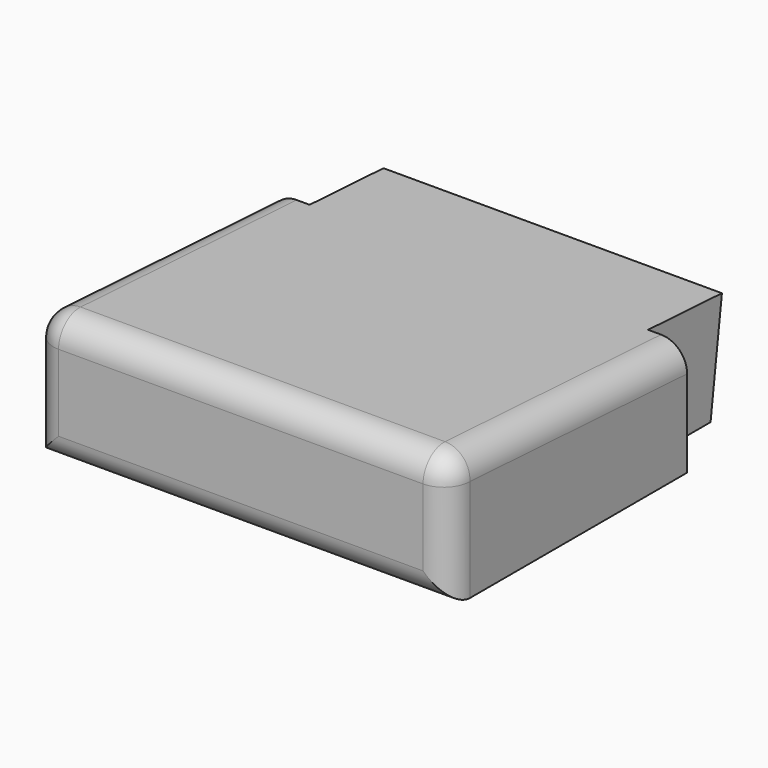
from build123d import *

# Parameters (mm, degrees)
F1_DEPTH     = 406.4
F2_T1_DEPTH  = 417.5993599931
F2_T3_DEPTH  = 355.6
F2_T5_DEPTH  = 163.5993599931
F2_T7_DEPTH  = 533.4
F2_T12_DEPTH = 25.4
F2_T18_DEPTH = 25.4
F3_W         = 89.2188286402
F3_H         = 154.1103798959
F4_DEPTH     = 127


# Not quite as in the source:
# - a fillet or chamfer that OpenCascade refuses, or shapes differently, is made with other operations: its cross-section is extruded or revolved along the edge and cut away or added
# - a feature names something its author has since deleted; it is built from what else it names


with BuildPart() as f1:
    # F0 (on Right) → F1 (new body)
    with BuildSketch(Plane.YZ):
        Polygon((113.1009757519, -66.1072761975), (126.957971921, 39.0469668974), (-253.4152170727, 60.8927238025), (-253.4152170727, -66.1072761975), align=None)
    extrude(amount=F1_DEPTH)

    # F2: fillet of radius 25.4 on 6 edges, made by hand

    # F2_s2 → F2_t1 (cut)
    with BuildSketch(Plane(origin=(0, 187.7009218342, -10.780120229), x_dir=(1, 0, 0), z_dir=(0, -0.9983548268, 0.0573379446))):
        with BuildLine():
            ThreePointArc((25.4, 46.2622370369), (7.4394877579, 38.822749279), (0, 20.8622370369))
            Line((0, 20.8622370369), (0, 46.2622370369))
            Line((0, 46.2622370369), (25.4, 46.2622370369))
        make_face()
        with BuildLine():
            ThreePointArc((381, 46.2622370369), (398.9605122421, 38.822749279), (406.4, 20.8622370369))
            Line((406.4, 20.8622370369), (406.4, 46.2622370369))
            Line((406.4, 46.2622370369), (381, 46.2622370369))
        make_face()
    extrude(amount=F2_T1_DEPTH, mode=Mode.SUBTRACT)

    # F2_s4 → F2_t3 (cut)
    with BuildSketch(Plane.YZ.offset(25.4)):
        with BuildLine():
            ThreePointArc((-226.558833279, 59.3502963952), (-245.4532194187, 52.4603288172), (-253.4152170727, 33.9920837956))
            Line((-253.4152170727, 33.9920837956), (-253.4152170727, 60.8927238025))
            Line((-253.4152170727, 60.8927238025), (-226.558833279, 59.3502963952))
        make_face()
    extrude(amount=F2_T3_DEPTH, mode=Mode.SUBTRACT)

    # F2_s6 → F2_t5 (cut)
    with BuildSketch(Plane.XY.offset(-129.6072761975)):
        with BuildLine():
            ThreePointArc((25.4, -253.4152170727), (7.4394877579, -245.9757293148), (0, -228.0152170727))
            Line((0, -228.0152170727), (0, -253.4152170727))
            Line((0, -253.4152170727), (25.4, -253.4152170727))
        make_face()
        with BuildLine():
            ThreePointArc((381, -253.4152170727), (398.9605122421, -245.9757293148), (406.4, -228.0152170727))
            Line((406.4, -228.0152170727), (406.4, -253.4152170727))
            Line((406.4, -253.4152170727), (381, -253.4152170727))
        make_face()
    extrude(amount=F2_T5_DEPTH, mode=Mode.SUBTRACT)

    # F2_s8 → F2_t7 (cut)
    with BuildSketch(Plane.YZ.offset(-63.5)):
        with BuildLine():
            ThreePointArc((-253.4152170727, -40.7072761975), (-245.9757293148, -58.6677884397), (-228.0152170727, -66.1072761975))
            Line((-228.0152170727, -66.1072761975), (-253.4152170727, -66.1072761975))
            Line((-253.4152170727, -66.1072761975), (-253.4152170727, -40.7072761975))
        make_face()
    extrude(amount=F2_T7_DEPTH, mode=Mode.SUBTRACT)


with BuildPart() as f2_tool10:
    # F2_s11 → F2_t12 (new body)
    with BuildSketch(Plane.YZ.offset(25.4)):
        Polygon((-228.0152170727, 33.9920837956), (-226.558833279, 59.3502963952), (-253.4152170727, 60.8927238025), (-253.4152170727, 33.9920837956), align=None)
    extrude(amount=-F2_T12_DEPTH)

    # F2_s13 → F2_t14 (revolve, cut)
    with BuildSketch(Plane(origin=(25.4, -228.0152170727, 33.9920837956), x_dir=(0, 0.6865355254, -0.7270962607), z_dir=(0, 0.7270962607, 0.6865355254))):
        with BuildLine():
            ThreePointArc((0, -25.4), (25.4, 0), (0, 25.4))
            Line((0, 25.4), (0, -25.4))
        make_face()
    revolve(axis=Axis((25.4, -228.0152170727, 33.9920837956), (-1, 0, 0)), mode=Mode.SUBTRACT)


with BuildPart() as f1_1:
    add(f1.part)

    # F2_t9: cut F2_tool10
    add(f2_tool10.part, mode=Mode.SUBTRACT)


with BuildPart() as f2_tool16:
    # F2_s17 → F2_t18 (new body)
    with BuildSketch(Plane.YZ.offset(381)):
        Polygon((-228.0152170727, 33.9920837956), (-226.558833279, 59.3502963952), (-253.4152170727, 60.8927238025), (-253.4152170727, 33.9920837956), align=None)
    extrude(amount=F2_T18_DEPTH)

    # F2_s19 → F2_t20 (revolve, cut)
    with BuildSketch(Plane(origin=(381, -228.0152170727, 33.9920837956), x_dir=(0, 0.6865355254, -0.7270962607), z_dir=(0, -0.7270962607, -0.6865355254))):
        with BuildLine():
            ThreePointArc((0, -25.4), (25.4, 0), (0, 25.4))
            Line((0, 25.4), (0, -25.4))
        make_face()
    revolve(axis=Axis((381, -228.0152170727, 33.9920837956), (1, 0, 0)), mode=Mode.SUBTRACT)


with BuildPart() as f1_2:
    add(f1_1.part)

    # F2_t15: cut F2_tool16
    add(f2_tool16.part, mode=Mode.SUBTRACT)

    # F3 (on face) → F4 (cut)
    with BuildSketch(Plane(origin=(0, 0, -66.1072761975), x_dir=(1, 0, 0), z_dir=(0, 0, -1))):
        with Locations((-6.5094143201, -113.9561656998)):
            Rectangle(F3_W, F3_H)
        with Locations((412.9094143201, -113.9561656998)):
            Rectangle(F3_W, F3_H)
    extrude(amount=-F4_DEPTH, mode=Mode.SUBTRACT)


solid = f1_2.part
